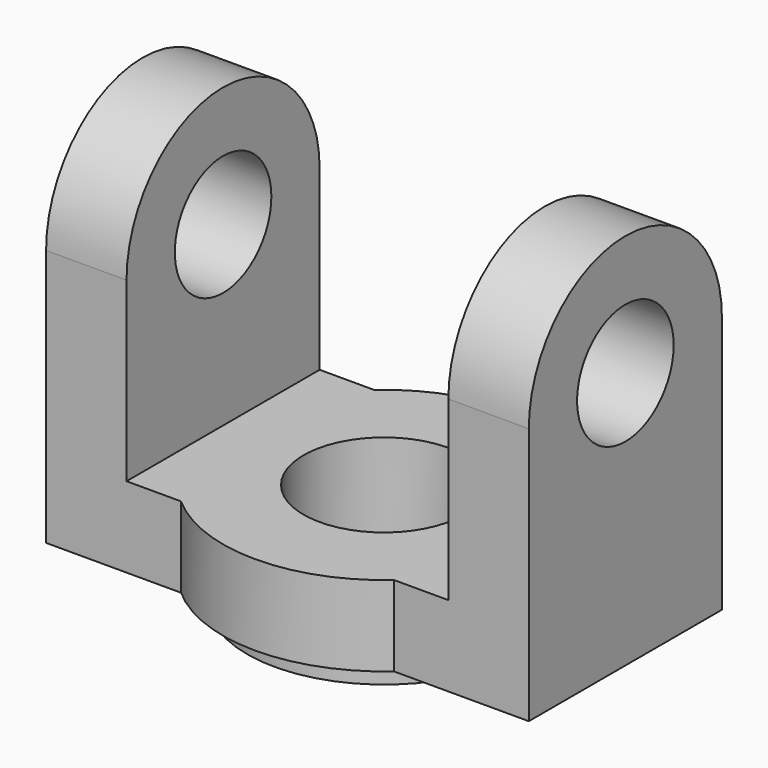
from build123d import *

# Parameters (mm, degrees)
F0_R          = 7.5
F1_DEPTH      = 30
F2_W          = 40
F2_H          = 48.8621479026
F3_DEPTH      = 15.001
F3_DEPTH_BACK = 15.001
F4_R          = 10
F5_DEPTH      = 32.001
F6_R          = 10
F7_DEPTH      = 10
F8_R          = 17
F8_R_2        = 10
F9_DEPTH      = 3


with BuildPart() as f1:
    # F0 (on Right) → F1 (new body, symmetric)
    with BuildSketch(Plane.YZ):
        with BuildLine():
            Line((-15, 0), (-15, -32))
            Line((-15, -32), (15, -32))
            Line((15, -32), (15, 0))
            ThreePointArc((15, 0), (0, 15), (-15, 0))
        make_face()
        Circle(F0_R, mode=Mode.SUBTRACT)
    extrude(amount=F1_DEPTH, both=True)

    # F2 (on Front) → F3 (cut, two sides)
    with BuildSketch(Plane.XZ) as f3_sk:
        with Locations((0, 2.4310739513)):
            Rectangle(F2_W, F2_H)
    extrude(amount=-F3_DEPTH, mode=Mode.SUBTRACT)
    extrude(f3_sk.sketch, amount=F3_DEPTH_BACK, mode=Mode.SUBTRACT)

    # F4 (on Top) → F5 (cut, through all)
    with BuildSketch(Plane.XY):
        Circle(F4_R)
    extrude(amount=-F5_DEPTH, mode=Mode.SUBTRACT)

    # F6 (on face) → F7 (join)
    with BuildSketch(Plane(origin=(0, 0, -32), x_dir=(1, 0, 0), z_dir=(0, 0, -1))):
        with BuildLine():
            ThreePointArc((13.2287565553, -15), (18.2287565553, -8.2287565553), (20, 0))
            ThreePointArc((20, 0), (18.2287565553, 8.2287565553), (13.2287565553, 15))
            Line((13.2287565553, 15), (-13.2287565553, 15))
            ThreePointArc((-13.2287565553, 15), (-20, 0), (-13.2287565553, -15))
            Line((-13.2287565553, -15), (13.2287565553, -15))
        make_face()
        Circle(F6_R, mode=Mode.SUBTRACT)
        with BuildLine():
            Line((-13.2287565553, 15), (13.2287565553, 15))
            ThreePointArc((13.2287565553, 15), (0, 20), (-13.2287565553, 15))
        make_face()
        with BuildLine():
            ThreePointArc((-13.2287565553, -15), (0, -20), (13.2287565553, -15))
            Line((13.2287565553, -15), (-13.2287565553, -15))
        make_face()
    extrude(amount=-F7_DEPTH)

    # F8 (on face) → F9 (join)
    with BuildSketch(Plane(origin=(0, 0, -32), x_dir=(1, 0, 0), z_dir=(0, 0, -1))):
        Circle(F8_R)
        Circle(F8_R_2, mode=Mode.SUBTRACT)
    extrude(amount=F9_DEPTH)


solid = f1.part
